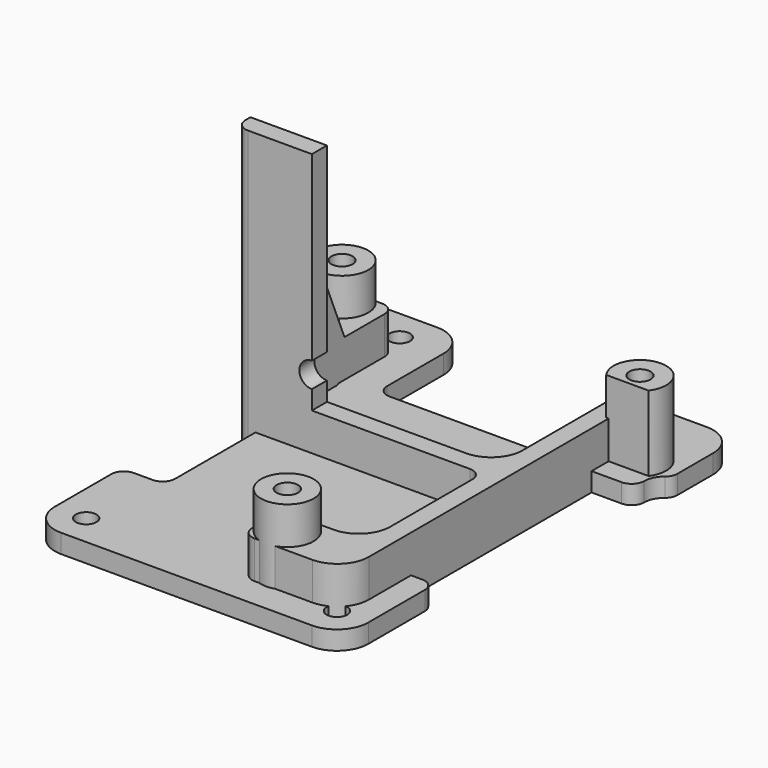
from build123d import *

# Parameters (mm, degrees)
F1_R      = 1.65
F2_DEPTH  = 3
F3_R      = 4.2
F4_DEPTH  = 12
F5_R      = 1.7
F6_DEPTH  = 15.001
F0_R      = 1.7
F7_DEPTH  = 2.6
F8_R      = 1.7
F9_DEPTH  = 9
F11_DEPTH = 36
F12_R     = 2
F13_DEPTH = 36.2510003725
F14_SIZE2 = 14.99999
F14_SIZE  = 35.99999


# Not quite as in the source:
# - a fillet or chamfer is up to 0.001 mm smaller than in the source, because OpenCascade refuses the exact size


with BuildPart() as f2:
    # F1 (on Top) → F2 (new body)
    with BuildSketch(Plane.XY):
        with BuildLine():
            Line((-25.0000003725, -20), (-25.0000003725, -31.2500003725))
            ThreePointArc((-25.0000003725, -31.2500003725), (-23.5355342785, -34.7855342785), (-20.0000003725, -36.2500003725))
            Line((-20.0000003725, -36.2500003725), (20.0000003725, -36.2500003725))
            ThreePointArc((20.0000003725, -36.2500003725), (23.5355342785, -34.7855342785), (25.0000003725, -31.2500003725))
            Line((25.0000003725, -31.2500003725), (25.0000003725, -20))
            ThreePointArc((25.0000003725, -20), (24.4142139349, -18.5857864376), (23.0000003725, -18))
            Line((23.0000003725, -18), (20, -18))
            ThreePointArc((20, -18), (18.5857864376, -17.4142135624), (18, -16))
            Line((18, -16), (18, 16))
            ThreePointArc((18, 16), (18.5857864376, 17.4142135624), (20, 18))
            Line((20, 18), (26, 18))
            ThreePointArc((26, 18), (27.4142135624, 18.5857864376), (28, 20))
            ThreePointArc((28, 20), (28.3258599148, 21.4184162865), (29.2380952381, 22.5523987206))
            ThreePointArc((29.2380952381, 22.5523987206), (29.7994708217, 23.2502340647), (30, 24.1231056256))
            Line((30, 24.1231056256), (30, 31.2500003725))
            ThreePointArc((30, 31.2500003725), (28.5355339059, 34.7855342785), (25, 36.2500003725))
            Line((25, 36.2500003725), (18, 36.2500003725))
            ThreePointArc((18, 36.2500003725), (14.4644660941, 34.7855342785), (13, 31.2500003725))
            Line((13, 31.2500003725), (13, 20))
            ThreePointArc((13, 20), (12.4142135624, 18.5857864376), (11, 18))
            Line((11, 18), (-11, 18))
            ThreePointArc((-11, 18), (-12.4142135624, 18.5857864376), (-13, 20))
            Line((-13, 20), (-13, 31.2500003725))
            ThreePointArc((-13, 31.2500003725), (-14.4644660941, 34.7855342785), (-18, 36.2500003725))
            Line((-18, 36.2500003725), (-20.0000003725, 36.2500003725))
            Line((-20.0000003725, 36.2500003725), (-25, 36.2500003725))
            ThreePointArc((-25, 36.2500003725), (-28.5355339059, 34.7855342785), (-30, 31.2500003725))
            Line((-30, 31.2500003725), (-30, 24.1231056256))
            ThreePointArc((-30, 24.1231056256), (-29.7994708217, 23.2502340647), (-29.2380952381, 22.5523987206))
            ThreePointArc((-29.2380952381, 22.5523987206), (-28.3258599148, 21.4184162865), (-28, 20))
            ThreePointArc((-28, 20), (-27.4142135624, 18.5857864376), (-26, 18))
            Line((-26, 18), (-20, 18))
            ThreePointArc((-20, 18), (-18.5857864376, 17.4142135624), (-18, 16))
            Line((-18, 16), (-18, -16))
            ThreePointArc((-18, -16), (-18.5857864376, -17.4142135624), (-20, -18))
            Line((-20, -18), (-23.0000003725, -18))
            ThreePointArc((-23.0000003725, -18), (-24.4142139349, -18.5857864376), (-25.0000003725, -20))
        make_face()
        with Locations((-20, -31.25)):
            Circle(F1_R, mode=Mode.SUBTRACT)
        with Locations((20, -31.25)):
            Circle(F1_R, mode=Mode.SUBTRACT)
        with Locations((-20, 31.25)):
            Circle(F1_R, mode=Mode.SUBTRACT)
        with Locations((20, 31.25)):
            Circle(F1_R, mode=Mode.SUBTRACT)
    extrude(amount=F2_DEPTH)

    # F3 (on face) → F4 (join)
    with BuildSketch(Plane.XY.offset(3)):
        with BuildLine():
            Line((20.8250925939, 21.4), (27.5749074061, 21.4))
            ThreePointArc((27.5749074061, 21.4), (24.2, 28.1), (20.8250925939, 21.4))
        make_face()
        with Locations((9, -27.4)):
            Circle(F3_R)
        with Locations((-24.2, 25)):
            Circle(F3_R)
    extrude(amount=F4_DEPTH)

    # F5 (on face) → F6 (cut, through all)
    with BuildSketch(Plane.XY.offset(15)):
        with Locations((-24.2, 25)):
            Circle(F5_R)
        with Locations((24.2, 23.9)):
            Circle(F5_R)
        with Locations((9, -27.4)):
            Circle(F5_R)
    extrude(amount=-F6_DEPTH, mode=Mode.SUBTRACT)

    # F0 (on Top) → F7 (cut)
    with BuildSketch(Plane.XY):
        Polygon((-26.95, 26.5877132403), (-26.95, 23.4122867597), (-24.2, 21.8245735195), (-21.45, 23.4122867597), (-21.45, 26.5877132403), (-24.2, 28.1754264805), align=None)
        with Locations((-24.2, 25)):
            Circle(F0_R, mode=Mode.SUBTRACT)
        Polygon((26.95, 22.3122867597), (26.95, 25.4877132403), (24.2, 27.0754264805), (21.45, 25.4877132403), (21.45, 22.3122867597), (24.2, 20.7245735195), align=None)
        with Locations((24.2, 23.9)):
            Circle(F0_R, mode=Mode.SUBTRACT)
        Polygon((11.75, -28.9877132403), (11.75, -25.8122867597), (9, -24.2245735195), (6.25, -25.8122867597), (6.25, -28.9877132403), (9, -30.5754264805), align=None)
        with Locations((9, -27.4)):
            Circle(F0_R, mode=Mode.SUBTRACT)
    extrude(amount=F7_DEPTH, mode=Mode.SUBTRACT)


with BuildPart() as f9:
    # F8 (on Top) → F9 (new body)
    with BuildSketch(Plane.XY):
        with BuildLine():
            ThreePointArc((-21.2, 2), (-20.6142135624, 0.5857864376), (-19.2, 0))
            Line((-19.2, 0), (16.2, 0))
            ThreePointArc((16.2, 0), (17.6142135624, -0.5857864376), (18.2, -2))
            Line((18.2, -2), (18.2, -18.4))
            ThreePointArc((18.2, -18.4), (16.7355339059, -21.9355339059), (13.2, -23.4))
            Line((13.2, -23.4), (7, -23.4))
            ThreePointArc((7, -23.4), (5.5857864376, -23.9857864376), (5, -25.4))
            Line((5, -25.4), (5, -29.4))
            ThreePointArc((5, -29.4), (5.5857864376, -30.8142135624), (7, -31.4))
            Line((7, -31.4), (16.2, -31.4))
            ThreePointArc((16.2, -31.4), (19.7355339059, -29.9355339059), (21.2, -26.4))
            Line((21.2, -26.4), (21.2, 21.6))
            Line((21.2, 21.6), (27.2, 21.6))
            Line((27.2, 21.6), (27.2, 26))
            ThreePointArc((27.2, 26), (26.6142135624, 27.4142135624), (25.2, 28))
            Line((25.2, 28), (20.2, 28))
            ThreePointArc((20.2, 28), (18.7857864376, 27.4142135624), (18.2, 26))
            Line((18.2, 26), (18.2, 8))
            ThreePointArc((18.2, 8), (16.7355339059, 4.4644660941), (13.2, 3))
            Line((13.2, 3), (-13.2, 3))
            ThreePointArc((-13.2, 3), (-16.7355339059, 4.4644660941), (-18.2, 8))
            Line((-18.2, 8), (-18.2, 18.8116944134))
            Line((-18.2, 18.8116944134), (-18.2, 26))
            ThreePointArc((-18.2, 26), (-18.7857864376, 27.4142135624), (-20.2, 28))
            Line((-20.2, 28), (-25.2, 28))
            ThreePointArc((-25.2, 28), (-26.6142135624, 27.4142135624), (-27.2, 26))
            Line((-27.2, 26), (-27.2, 24))
            ThreePointArc((-27.2, 24), (-26.6142135624, 22.5857864376), (-25.2, 22))
            Line((-25.2, 22), (-23.2, 22))
            ThreePointArc((-23.2, 22), (-21.7857864376, 21.4142135624), (-21.2, 20))
            Line((-21.2, 20), (-21.2, 2))
        make_face()
        with Locations((9, -27.4)):
            Circle(F8_R, mode=Mode.SUBTRACT)
        with Locations((-24.2, 25)):
            Circle(F8_R, mode=Mode.SUBTRACT)
        with Locations((24.2, 23.9)):
            Circle(F8_R, mode=Mode.SUBTRACT)
    extrude(amount=F9_DEPTH)

    # F10 (on face) → F11 (join)
    with BuildSketch(Plane.XY.offset(9)):
        with BuildLine():
            Line((-9, 0), (-9, 3))
            Line((-9, 3), (-13.2, 3))
            ThreePointArc((-13.2, 3), (-16.7355339059, 4.4644660941), (-18.2, 8))
            Line((-18.2, 8), (-18.2, 18))
            Line((-18.2, 18), (-21.2, 18))
            Line((-21.2, 18), (-21.2, 2))
            ThreePointArc((-21.2, 2), (-20.6142135624, 0.5857864376), (-19.2, 0))
            Line((-19.2, 0), (-9, 0))
        make_face()
    extrude(amount=F11_DEPTH)

    # F12 (on face) → F13 (cut, through all)
    with BuildSketch(Plane.XZ):
        with Locations((-9, 14)):
            Circle(F12_R)
    extrude(amount=-F13_DEPTH, mode=Mode.SUBTRACT)

    # F14 (size 36 and 15 in the source; OpenCascade refuses exactly that, so slightly less here)
    f14_edges = [f9.edges().sort_by_distance(p)[0] for p in [
        (-19.7, 18, 45),
    ]]
    f14_side = f9.faces().sort_by_distance((-19.7, 18, 27))[0]
    chamfer(f14_edges, length=F14_SIZE, length2=F14_SIZE2, reference=f14_side)


solid = Compound([f2.part, f9.part])
